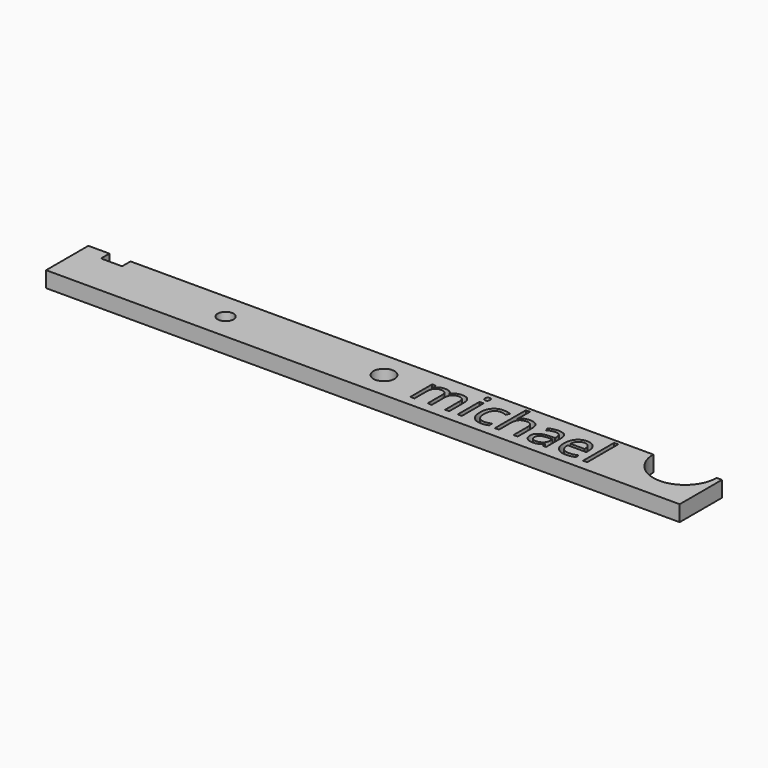
from build123d import *

# Parameters (mm, degrees)
F0_R         = 1.5
F0_R_2       = 2
F1_DEPTH     = 3
F2_TEXT_SIZE = 9.6507357537
F3_DEPTH     = 25


# Not quite as in the source:
# - Text() gives the source's letters only with a copy of the font that has no kerning and outlines rounded to 1/6400 em; it was checked with that copy


with BuildPart() as f1:
    # F0 (on Top) → F1 (new body)
    with BuildSketch(Plane.XY):
        with BuildLine():
            Line((-60, -5), (-4.8989794856, -5))
            ThreePointArc((-4.8989794856, -5), (-7, 0), (-4.8989794856, 5))
            Line((-4.8989794856, 5), (-52, 5))
            Line((-52, 5), (-52, 3))
            Line((-52, 3), (-56, 3))
            Line((-56, 3), (-56, 5))
            Line((-56, 5), (-60, 5))
            Line((-60, 5), (-60, -5))
        make_face()
        with Locations((-30, 0)):
            Circle(F0_R, mode=Mode.SUBTRACT)
        with BuildLine():
            Line((4.8989794856, -5), (60, -5))
            Line((60, -5), (60, 5))
            Line((60, 5), (59, 5))
            ThreePointArc((59, 5), (53, -1), (47, 5))
            Line((47, 5), (4.8989794856, 5))
            ThreePointArc((4.8989794856, 5), (6.4534043883, 2.7117470016), (7, 0))
            ThreePointArc((7, 0), (6.4534043883, -2.7117470016), (4.8989794856, -5))
        make_face()
        with BuildLine():
            Line((-4.8989794856, -5), (4.8989794856, -5))
            ThreePointArc((4.8989794856, -5), (6.4534043883, -2.7117470016), (7, 0))
            ThreePointArc((7, 0), (6.4534043883, 2.7117470016), (4.8989794856, 5))
            Line((4.8989794856, 5), (-4.8989794856, 5))
            ThreePointArc((-4.8989794856, 5), (-7, 0), (-4.8989794856, -5))
        make_face()
        Circle(F0_R_2, mode=Mode.SUBTRACT)
    extrude(amount=F1_DEPTH)

    # F2 (on face) → F3 (cut)
    with BuildSketch(Plane.XY.offset(3)):
        with Locations((6.5920464694, -3.044315381)):
            Text('michael', F2_TEXT_SIZE, font='Open Sans', text_align=(TextAlign.LEFT, TextAlign.BOTTOM))
    extrude(amount=-F3_DEPTH, mode=Mode.SUBTRACT)


solid = f1.part
